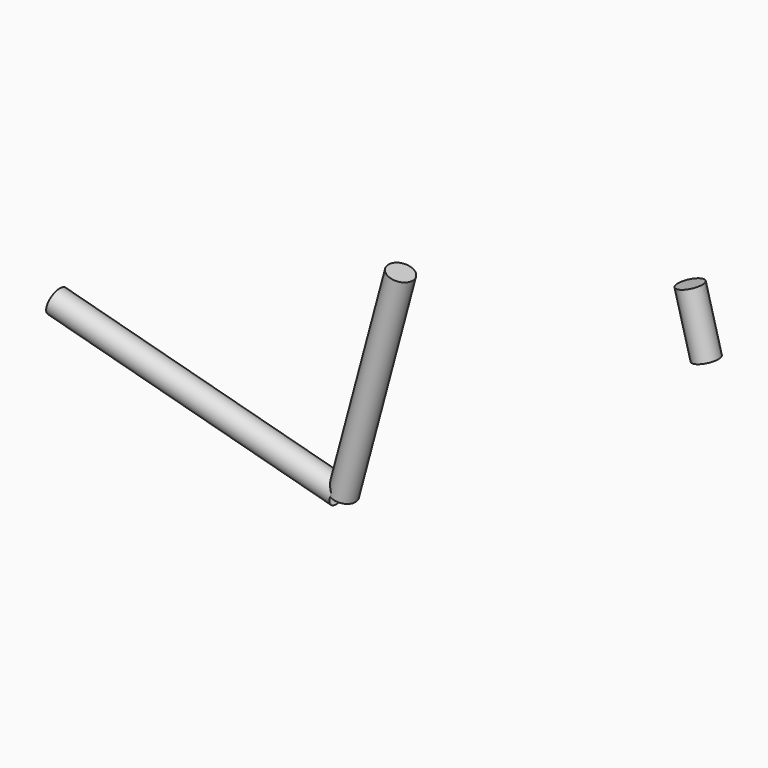
from build123d import *


with BuildPart() as f1:
    # F0 (on Front) → F1 (revolve)
    with BuildSketch(Plane.XZ):
        with BuildLine():
            ThreePointArc((-25.4, 0), (-25.1225509895, 3.7439860819), (-24.2962652141, 7.4061796256))
            Line((-24.2962652141, 7.4061796256), (-582.2543799602, 156.9106058822))
            Line((-582.2543799602, 156.9106058822), (-588.8283837058, 132.3760898945))
            Line((-588.8283837058, 132.3760898945), (-12.7, -21.9970452561))
            ThreePointArc((-12.7, -21.9970452561), (-21.9970452561, -12.7), (-25.4, 0))
        make_face()
    revolve(axis=Axis((-173.5640761914, 0, 47.402369033), (0.9659258263, 0, -0.2588190451)))

    # F0 (on Front) → F2 (revolve)
    with BuildSketch(Plane.XZ):
        with BuildLine():
            ThreePointArc((12.7, 21.9970452561), (21.9970452561, 12.7), (25.4, 0))
            ThreePointArc((25.4, 0), (25.2355357256, -2.8857818079), (24.7442727053, -5.7341929063))
            Line((24.7442727053, -5.7341929063), (25.594513093, -5.9620141315))
            Line((25.594513093, -5.9620141315), (119.2280824033, 343.4832238284))
            Line((119.2280824033, 343.4832238284), (130.6145908998, 385.9782520583))
            Line((130.6145908998, 385.9782520583), (102.2845720799, 378.3872463939))
            Line((102.2845720799, 378.3872463939), (7.6340008509, 25.1465056018))
            Line((7.6340008509, 25.1465056018), (13.1480074912, 23.6690319755))
            Line((13.1480074912, 23.6690319755), (12.7, 21.9970452561))
        make_face()
        Polygon((117.4665834086, 435.0472840338), (102.2845720799, 378.3872463939), (130.6145908998, 385.9782520583), (142.0010993964, 428.4732802882), align=None)
    revolve(axis=Axis((44.8725568947, 0, 164.1226887577), (-0.2588190451, 0, -0.9659258263)))


with BuildPart() as f3:
    # F0 (on Front) → F3 (revolve)
    with BuildSketch(Plane.XZ):
        Polygon((698.1954604907, 538.0610877045), (708.0564661091, 501.2593137229), (714.6304698547, 476.7247977351), (739.1649858425, 483.2988014808), (722.7299764784, 544.6350914501), align=None)
        Polygon((688.3344548723, 574.8628616861), (698.1954604907, 538.0610877045), (722.7299764784, 544.6350914501), (706.2949671144, 605.9713814195), (681.7604511267, 599.3973776739), align=None)
    revolve(axis=Axis((729.8902228261, 0, 517.9126882861), (0.2588190451, 0, -0.9659258263)))


solid = Compound([f1.part, f3.part])
